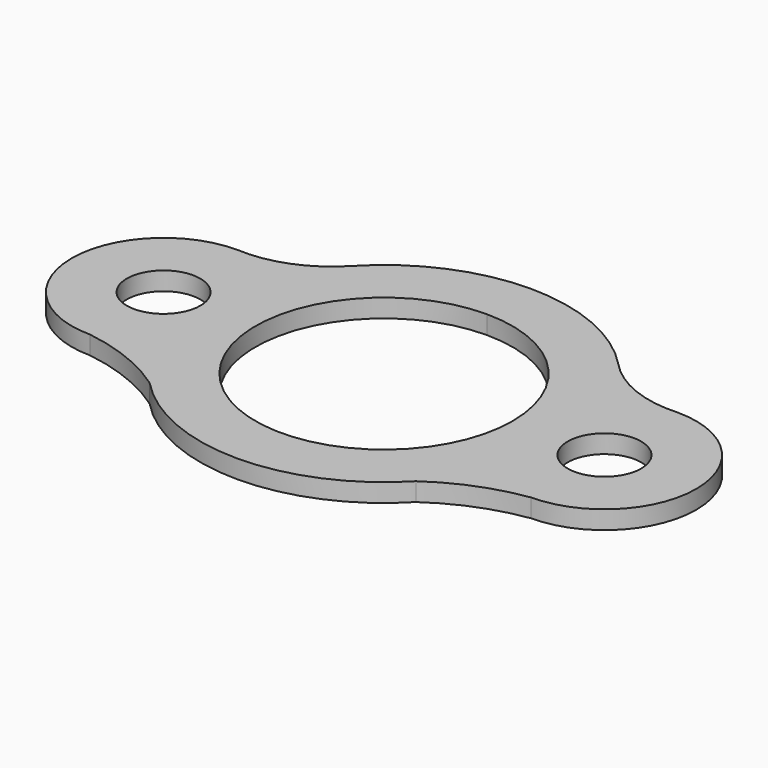
from build123d import *

# Parameters (mm, degrees)
F0_R     = 12.7
F1_DEPTH = 6.35


# Not quite as in the source:
# - a feature names something its author has since deleted; it is built from what else it names


with BuildPart() as f1:
    # F0 (on Top) → F1 (new body)
    with BuildSketch(Plane.XY):
        with BuildLine():
            ThreePointArc((46.002574141, 43.7722877218), (25.0270826273, 58.3600474226), (0, 63.5))
            ThreePointArc((0, 63.5), (-25.0270826273, 58.3600474226), (-46.002574141, 43.7722877218))
            ThreePointArc((-46.002574141, 43.7722877218), (-59.7549711548, 34.379485063), (-76.2, 31.75))
            ThreePointArc((-76.2, 31.75), (-107.95, 0), (-76.2, -31.75))
            ThreePointArc((-76.2, -31.75), (-60.3918607808, -35.9792161379), (-46.002574141, -43.7722877218))
            ThreePointArc((-46.002574141, -43.7722877218), (0, -63.5), (46.002574141, -43.7722877218))
            ThreePointArc((46.002574141, -43.7722877218), (60.3918607808, -35.9792161379), (76.2, -31.75))
            ThreePointArc((76.2, -31.75), (107.95, 0), (76.2, 31.75))
            ThreePointArc((76.2, 31.75), (59.7549711548, 34.379485063), (46.002574141, 43.7722877218))
        make_face()
        with Locations((-76.2, 0)):
            Circle(F0_R, mode=Mode.SUBTRACT)
        with BuildLine():
            ThreePointArc((0, 44.45), (31.4308964237, 31.4308964237), (44.45, 0))
            ThreePointArc((44.45, 0), (-31.4308964237, -31.4308964237), (0, 44.45))
        make_face(mode=Mode.SUBTRACT)
        with Locations((76.2, 0)):
            Circle(F0_R, mode=Mode.SUBTRACT)
    extrude(amount=F1_DEPTH)


solid = f1.part
